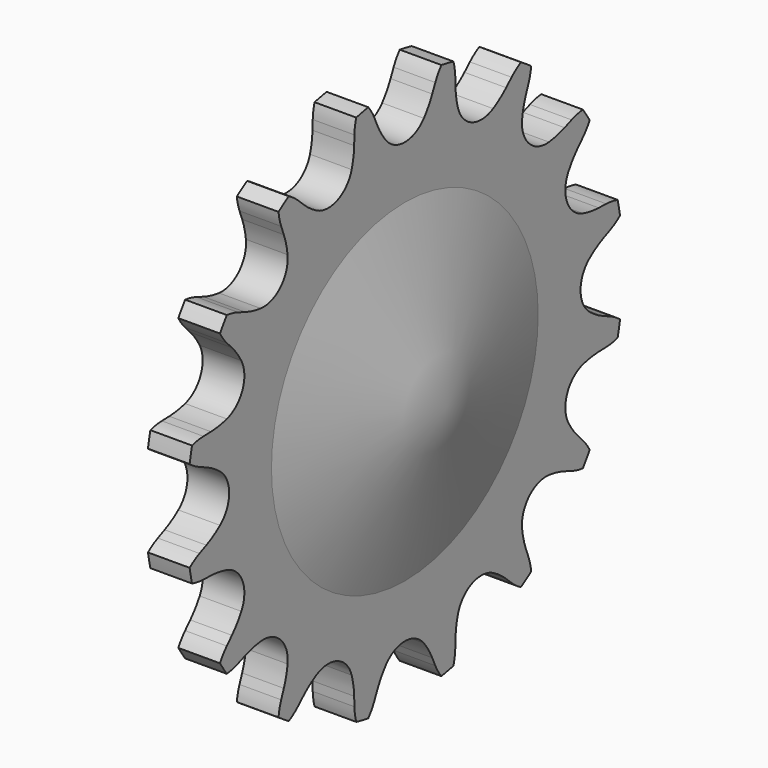
from build123d import *

# Parameters (mm, degrees)
F0_W     = 12.7
F0_H     = 25.4
F0_H_2   = 38.1
F2_R     = 25.4
F3_DEPTH = 25.401
F4_R     = 50.8
F4_R_2   = 25.4
F5_DEPTH = 12.7
F6_R     = 25.4
F7_DEPTH = 12.7


# Not quite as in the source:
# - a fillet or chamfer that OpenCascade refuses, or shapes differently, is made with other operations: its cross-section is extruded or revolved along the edge and cut away or added


with BuildPart() as f1:
    # F0 (on Front) → F1 (revolve)
    with BuildSketch(Plane.XZ):
        with Locations((-13.1482736327, -38.1)):
            Rectangle(F0_W, F0_H)
        with Locations((-25.8482736327, 69.85)):
            Rectangle(F0_W, F0_H_2)
        with Locations((-13.1482736327, 38.1)):
            Rectangle(F0_W, F0_H)
        with Locations((-25.8482736327, -38.1)):
            Rectangle(F0_W, F0_H)
        with Locations((-25.8482736327, 38.1)):
            Rectangle(F0_W, F0_H)
        with Locations((-25.8482736327, -69.85)):
            Rectangle(F0_W, F0_H_2)
    revolve(axis=Axis((0.2396887807, 0, 0), (1, 0, 0)))

    # F2 (on face) → F3 (intersect, through all)
    with BuildSketch(Plane(origin=(-32.1982736327, 0, 0), x_dir=(0, -1, 0), z_dir=(-1, 0, 0))):
        with BuildLine():
            ThreePointArc((-7.2342121166, 70.3939309414), (-8.9992882213, 72.9030522861), (-10.4336039265, 75.6148638643))
            Line((-10.4336039265, 75.6148638643), (-11.603456176, 78.2118395592))
            ThreePointArc((-11.603456176, 78.2118395592), (-12.6397989195, 80.1661730867), (-13.9183429757, 81.97137416))
            ThreePointArc((-13.9183429757, 81.97137416), (-16.2207090683, 81.5470112891), (-18.5102146175, 81.057994101))
            ThreePointArc((-18.5102146175, 81.057994101), (-19.0006147597, 78.9009281495), (-19.2101795467, 76.6987682056))
            Line((-19.2101795467, 76.6987682056), (-19.2971625233, 73.8517924404))
            ThreePointArc((-19.2971625233, 73.8517924404), (-19.5845320839, 70.7975163701), (-20.255050602, 67.803925133))
            ThreePointArc((-20.255050602, 67.803925133), (-25.6107042359, 61.8297095082), (-33.6221316187, 62.2670988866))
            ThreePointArc((-33.6221316187, 62.2670988866), (-36.2130484736, 63.9097593594), (-38.5759487594, 65.8662577153))
            Line((-38.5759487594, 65.8662577153), (-40.6505708816, 67.8178673321))
            ThreePointArc((-40.6505708816, 67.8178673321), (-42.3559177932, 69.2268448797), (-44.2279590209, 70.4053555754))
            ThreePointArc((-44.2279590209, 70.4053555754), (-46.1926712902, 69.1322180458), (-48.1207598307, 67.8042692327))
            ThreePointArc((-48.1207598307, 67.8042692327), (-47.7483570826, 65.6237321402), (-47.0992395741, 63.5090046687))
            Line((-47.0992395741, 63.5090046687), (-46.0901109083, 60.8454550856))
            ThreePointArc((-46.0901109083, 60.8454550856), (-45.1867849136, 57.9137003678), (-44.6606654789, 54.8913863673))
            ThreePointArc((-44.6606654789, 54.8913863673), (-47.3224109134, 47.3224109134), (-54.8913863673, 44.6606654789))
            ThreePointArc((-54.8913863673, 44.6606654789), (-57.9137003678, 45.1867849136), (-60.8454550856, 46.0901109083))
            Line((-60.8454550856, 46.0901109083), (-63.5090046687, 47.0992395741))
            ThreePointArc((-63.5090046687, 47.0992395741), (-65.6237321402, 47.7483570826), (-67.8042692327, 48.1207598307))
            ThreePointArc((-67.8042692327, 48.1207598307), (-69.1322180458, 46.1926712902), (-70.4053555754, 44.2279590209))
            ThreePointArc((-70.4053555754, 44.2279590209), (-69.2268448797, 42.3559177932), (-67.8178673321, 40.6505708816))
            Line((-67.8178673321, 40.6505708816), (-65.8662577153, 38.5759487594))
            ThreePointArc((-65.8662577153, 38.5759487594), (-63.9097593594, 36.2130484736), (-62.2670988866, 33.6221316187))
            ThreePointArc((-62.2670988866, 33.6221316187), (-61.8297095082, 25.6107042359), (-67.803925133, 20.255050602))
            ThreePointArc((-67.803925133, 20.255050602), (-70.7975163701, 19.5845320839), (-73.8517924404, 19.2971625233))
            Line((-73.8517924404, 19.2971625233), (-76.6987682056, 19.2101795467))
            ThreePointArc((-76.6987682056, 19.2101795467), (-78.9009281495, 19.0006147597), (-81.057994101, 18.5102146175))
            ThreePointArc((-81.057994101, 18.5102146175), (-81.5470112891, 16.2207090683), (-81.97137416, 13.9183429757))
            ThreePointArc((-81.97137416, 13.9183429757), (-80.1661730867, 12.6397989195), (-78.2118395592, 11.603456176))
            Line((-78.2118395592, 11.603456176), (-75.6148638643, 10.4336039265))
            ThreePointArc((-75.6148638643, 10.4336039265), (-72.9030522861, 8.9992882213), (-70.3939309414, 7.2342121166))
            ThreePointArc((-70.3939309414, 7.2342121166), (-66.923995318, 0), (-70.3939309414, -7.2342121166))
            ThreePointArc((-70.3939309414, -7.2342121166), (-72.9030522861, -8.9992882213), (-75.6148638643, -10.4336039265))
            Line((-75.6148638643, -10.4336039265), (-78.2118395592, -11.603456176))
            ThreePointArc((-78.2118395592, -11.603456176), (-80.1661730867, -12.6397989195), (-81.97137416, -13.9183429757))
            ThreePointArc((-81.97137416, -13.9183429757), (-81.5470112891, -16.2207090683), (-81.057994101, -18.5102146175))
            ThreePointArc((-81.057994101, -18.5102146175), (-78.9009281495, -19.0006147597), (-76.6987682056, -19.2101795467))
            Line((-76.6987682056, -19.2101795467), (-73.8517924404, -19.2971625233))
            ThreePointArc((-73.8517924404, -19.2971625233), (-70.7975163701, -19.5845320839), (-67.803925133, -20.255050602))
            ThreePointArc((-67.803925133, -20.255050602), (-61.8297095082, -25.6107042359), (-62.2670988866, -33.6221316187))
            ThreePointArc((-62.2670988866, -33.6221316187), (-63.9097593594, -36.2130484736), (-65.8662577153, -38.5759487594))
            Line((-65.8662577153, -38.5759487594), (-67.8178673321, -40.6505708816))
            ThreePointArc((-67.8178673321, -40.6505708816), (-69.2268448797, -42.3559177932), (-70.4053555754, -44.2279590209))
            ThreePointArc((-70.4053555754, -44.2279590209), (-69.1322180458, -46.1926712902), (-67.8042692327, -48.1207598307))
            ThreePointArc((-67.8042692327, -48.1207598307), (-65.6237321402, -47.7483570826), (-63.5090046687, -47.0992395741))
            Line((-63.5090046687, -47.0992395741), (-60.8454550856, -46.0901109083))
            ThreePointArc((-60.8454550856, -46.0901109083), (-57.9137003678, -45.1867849136), (-54.8913863673, -44.6606654789))
            ThreePointArc((-54.8913863673, -44.6606654789), (-47.3224109134, -47.3224109134), (-44.6606654789, -54.8913863673))
            ThreePointArc((-44.6606654789, -54.8913863673), (-45.1867849136, -57.9137003678), (-46.0901109083, -60.8454550856))
            Line((-46.0901109083, -60.8454550856), (-47.0992395741, -63.5090046687))
            ThreePointArc((-47.0992395741, -63.5090046687), (-47.7483570826, -65.6237321402), (-48.1207598307, -67.8042692327))
            ThreePointArc((-48.1207598307, -67.8042692327), (-46.1926712902, -69.1322180458), (-44.2279590209, -70.4053555754))
            ThreePointArc((-44.2279590209, -70.4053555754), (-42.3559177932, -69.2268448797), (-40.6505708816, -67.8178673321))
            Line((-40.6505708816, -67.8178673321), (-38.5759487594, -65.8662577153))
            ThreePointArc((-38.5759487594, -65.8662577153), (-36.2130484736, -63.9097593594), (-33.6221316187, -62.2670988866))
            ThreePointArc((-33.6221316187, -62.2670988866), (-25.6107042359, -61.8297095082), (-20.255050602, -67.803925133))
            ThreePointArc((-20.255050602, -67.803925133), (-19.5845320839, -70.7975163701), (-19.2971625233, -73.8517924404))
            Line((-19.2971625233, -73.8517924404), (-19.2101795467, -76.6987682056))
            ThreePointArc((-19.2101795467, -76.6987682056), (-19.0006147597, -78.9009281495), (-18.5102146175, -81.057994101))
            ThreePointArc((-18.5102146175, -81.057994101), (-16.2207090683, -81.5470112891), (-13.9183429757, -81.97137416))
            ThreePointArc((-13.9183429757, -81.97137416), (-12.6397989195, -80.1661730867), (-11.603456176, -78.2118395592))
            Line((-11.603456176, -78.2118395592), (-10.4336039265, -75.6148638643))
            ThreePointArc((-10.4336039265, -75.6148638643), (-8.9992882213, -72.9030522861), (-7.2342121166, -70.3939309414))
            ThreePointArc((-7.2342121166, -70.3939309414), (0, -66.923995318), (7.2342121166, -70.3939309414))
            ThreePointArc((7.2342121166, -70.3939309414), (8.9992882213, -72.9030522861), (10.4336039265, -75.6148638643))
            Line((10.4336039265, -75.6148638643), (11.603456176, -78.2118395592))
            ThreePointArc((11.603456176, -78.2118395592), (12.6397989195, -80.1661730867), (13.9183429757, -81.97137416))
            ThreePointArc((13.9183429757, -81.97137416), (16.2207090683, -81.5470112891), (18.5102146175, -81.057994101))
            ThreePointArc((18.5102146175, -81.057994101), (19.0006147597, -78.9009281495), (19.2101795467, -76.6987682056))
            Line((19.2101795467, -76.6987682056), (19.2971625233, -73.8517924404))
            ThreePointArc((19.2971625233, -73.8517924404), (19.5845320839, -70.7975163701), (20.255050602, -67.803925133))
            ThreePointArc((20.255050602, -67.803925133), (25.6107042359, -61.8297095082), (33.6221316187, -62.2670988866))
            ThreePointArc((33.6221316187, -62.2670988866), (36.2130484736, -63.9097593594), (38.5759487594, -65.8662577153))
            Line((38.5759487594, -65.8662577153), (40.6505708816, -67.8178673321))
            ThreePointArc((40.6505708816, -67.8178673321), (42.3559177932, -69.2268448797), (44.2279590209, -70.4053555754))
            ThreePointArc((44.2279590209, -70.4053555754), (46.1926712902, -69.1322180458), (48.1207598307, -67.8042692327))
            ThreePointArc((48.1207598307, -67.8042692327), (47.7483570826, -65.6237321402), (47.0992395741, -63.5090046687))
            Line((47.0992395741, -63.5090046687), (46.0901109083, -60.8454550856))
            ThreePointArc((46.0901109083, -60.8454550856), (45.1867849136, -57.9137003678), (44.6606654789, -54.8913863673))
            ThreePointArc((44.6606654789, -54.8913863673), (47.3224109134, -47.3224109134), (54.8913863673, -44.6606654789))
            ThreePointArc((54.8913863673, -44.6606654789), (57.9137003678, -45.1867849136), (60.8454550856, -46.0901109083))
            Line((60.8454550856, -46.0901109083), (63.5090046687, -47.0992395741))
            ThreePointArc((63.5090046687, -47.0992395741), (65.6237321402, -47.7483570826), (67.8042692327, -48.1207598307))
            ThreePointArc((67.8042692327, -48.1207598307), (69.1322180458, -46.1926712902), (70.4053555754, -44.2279590209))
            ThreePointArc((70.4053555754, -44.2279590209), (69.2268448797, -42.3559177932), (67.8178673321, -40.6505708816))
            Line((67.8178673321, -40.6505708816), (65.8662577153, -38.5759487594))
            ThreePointArc((65.8662577153, -38.5759487594), (63.9097593594, -36.2130484736), (62.2670988866, -33.6221316187))
            ThreePointArc((62.2670988866, -33.6221316187), (61.8297095082, -25.6107042359), (67.803925133, -20.255050602))
            ThreePointArc((67.803925133, -20.255050602), (70.7975163701, -19.5845320839), (73.8517924404, -19.2971625233))
            Line((73.8517924404, -19.2971625233), (76.6987682056, -19.2101795467))
            ThreePointArc((76.6987682056, -19.2101795467), (78.9009281495, -19.0006147597), (81.057994101, -18.5102146175))
            ThreePointArc((81.057994101, -18.5102146175), (81.5470112891, -16.2207090683), (81.97137416, -13.9183429757))
            ThreePointArc((81.97137416, -13.9183429757), (80.1661730867, -12.6397989195), (78.2118395592, -11.603456176))
            Line((78.2118395592, -11.603456176), (75.6148638643, -10.4336039265))
            ThreePointArc((75.6148638643, -10.4336039265), (72.9030522861, -8.9992882213), (70.3939309414, -7.2342121166))
            ThreePointArc((70.3939309414, -7.2342121166), (66.923995318, 0), (70.3939309414, 7.2342121166))
            ThreePointArc((70.3939309414, 7.2342121166), (72.9030522861, 8.9992882213), (75.6148638643, 10.4336039265))
            Line((75.6148638643, 10.4336039265), (78.2118395592, 11.603456176))
            ThreePointArc((78.2118395592, 11.603456176), (80.1661730867, 12.6397989195), (81.97137416, 13.9183429757))
            ThreePointArc((81.97137416, 13.9183429757), (81.5470112891, 16.2207090683), (81.057994101, 18.5102146175))
            ThreePointArc((81.057994101, 18.5102146175), (78.9009281495, 19.0006147597), (76.6987682056, 19.2101795467))
            Line((76.6987682056, 19.2101795467), (73.8517924404, 19.2971625233))
            ThreePointArc((73.8517924404, 19.2971625233), (70.7975163701, 19.5845320839), (67.803925133, 20.255050602))
            ThreePointArc((67.803925133, 20.255050602), (61.8297095082, 25.6107042359), (62.2670988866, 33.6221316187))
            ThreePointArc((62.2670988866, 33.6221316187), (63.9097593594, 36.2130484736), (65.8662577153, 38.5759487594))
            Line((65.8662577153, 38.5759487594), (67.8178673321, 40.6505708816))
            ThreePointArc((67.8178673321, 40.6505708816), (69.2268448797, 42.3559177932), (70.4053555754, 44.2279590209))
            ThreePointArc((70.4053555754, 44.2279590209), (69.1322180458, 46.1926712902), (67.8042692327, 48.1207598307))
            ThreePointArc((67.8042692327, 48.1207598307), (65.6237321402, 47.7483570826), (63.5090046687, 47.0992395741))
            Line((63.5090046687, 47.0992395741), (60.8454550856, 46.0901109083))
            ThreePointArc((60.8454550856, 46.0901109083), (57.9137003678, 45.1867849136), (54.8913863673, 44.6606654789))
            ThreePointArc((54.8913863673, 44.6606654789), (47.3224109134, 47.3224109134), (44.6606654789, 54.8913863673))
            ThreePointArc((44.6606654789, 54.8913863673), (45.1867849136, 57.9137003678), (46.0901109083, 60.8454550856))
            Line((46.0901109083, 60.8454550856), (47.0992395741, 63.5090046687))
            ThreePointArc((47.0992395741, 63.5090046687), (47.7483570826, 65.6237321402), (48.1207598307, 67.8042692327))
            ThreePointArc((48.1207598307, 67.8042692327), (46.1926712902, 69.1322180458), (44.2279590209, 70.4053555754))
            ThreePointArc((44.2279590209, 70.4053555754), (42.3559177932, 69.2268448797), (40.6505708816, 67.8178673321))
            Line((40.6505708816, 67.8178673321), (38.5759487594, 65.8662577153))
            ThreePointArc((38.5759487594, 65.8662577153), (36.2130484736, 63.9097593594), (33.6221316187, 62.2670988866))
            ThreePointArc((33.6221316187, 62.2670988866), (25.6107042359, 61.8297095082), (20.255050602, 67.803925133))
            ThreePointArc((20.255050602, 67.803925133), (19.5845320839, 70.7975163701), (19.2971625233, 73.8517924404))
            Line((19.2971625233, 73.8517924404), (19.2101795467, 76.6987682056))
            ThreePointArc((19.2101795467, 76.6987682056), (19.0006147597, 78.9009281495), (18.5102146175, 81.057994101))
            ThreePointArc((18.5102146175, 81.057994101), (16.2207090683, 81.5470112891), (13.9183429757, 81.97137416))
            ThreePointArc((13.9183429757, 81.97137416), (12.6397989195, 80.1661730867), (11.603456176, 78.2118395592))
            Line((11.603456176, 78.2118395592), (10.4336039265, 75.6148638643))
            ThreePointArc((10.4336039265, 75.6148638643), (8.9992882213, 72.9030522861), (7.2342121166, 70.3939309414))
            ThreePointArc((7.2342121166, 70.3939309414), (0, 66.923995318), (-7.2342121166, 70.3939309414))
        make_face()
        Circle(F2_R, mode=Mode.SUBTRACT)
    extrude(amount=-F3_DEPTH, mode=Mode.INTERSECT)

    # F4 (on face) → F5 (join)
    with BuildSketch(Plane.YZ.offset(-6.7982736327)):
        Circle(F4_R)
        Circle(F4_R_2, mode=Mode.SUBTRACT)
        Circle(F4_R_2)
    extrude(amount=-F5_DEPTH)

    # F6 (on face) → F7 (join)
    with BuildSketch(Plane(origin=(-32.1982736327, 0, 0), x_dir=(0, -1, 0), z_dir=(-1, 0, 0))):
        Circle(F6_R)
        Polygon((-12.7, -6.35), (-12.7, 6.35), (-6.35, 6.35), (-6.35, 12.7), (6.35, 12.7), (6.35, 6.35), (12.7, 6.35), (12.7, -6.35), (6.35, -6.35), (6.35, -12.7), (-6.35, -12.7), (-6.35, -6.35), align=None, mode=Mode.SUBTRACT)
    extrude(amount=-F7_DEPTH)

    # F8: chamfer of 12.7 x 50.8 on 1 edges, made by hand


with BuildPart() as f8_tool2:
    # F8_s3 → F8_t4 (revolve)
    with BuildSketch(Plane.XZ):
        Polygon((-6.7982736327, 0), (-19.4982736327, -50.8), (-6.7982736327, -50.8), align=None)
    revolve(axis=Axis((-6.7982736327, 0, 0), (1, 0, 0)))

    split(bisect_by=Plane.YZ.offset(-19.4982736327), keep=Keep.TOP)


with BuildPart() as f1_1:
    add(f1.part)

    # F8_t1: cut F8_tool2
    add(f8_tool2.part, mode=Mode.SUBTRACT)


solid = f1_1.part
